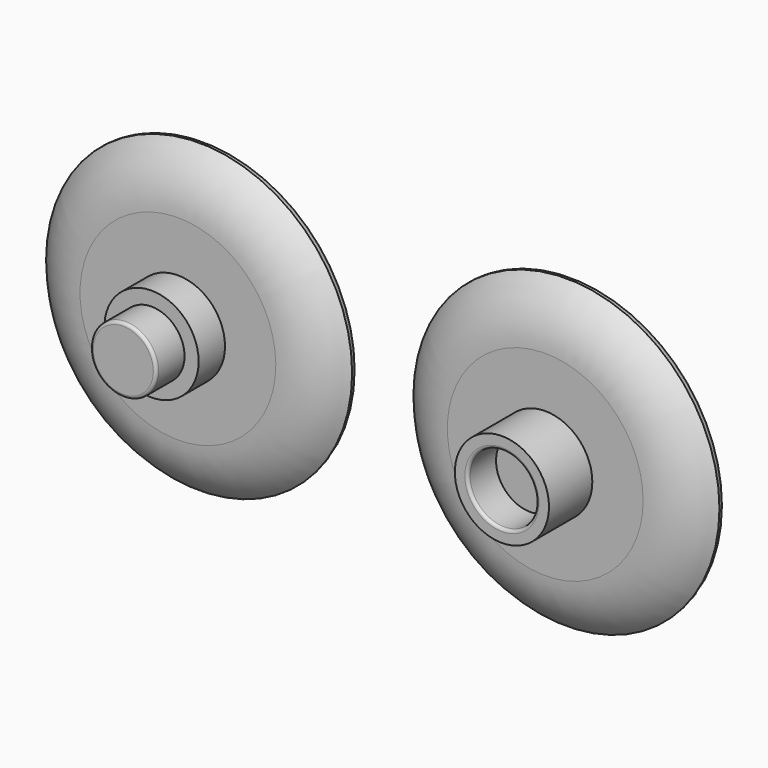
from build123d import *

# Parameters (mm, degrees)
F0_R      = 13
F1_DEPTH  = 3
F2_R      = 4
F3_DEPTH  = 2.8
F4_R      = 2.8
F5_DEPTH  = 3
F6_R      = 13
F7_DEPTH  = 3
F8_R      = 4
F9_DEPTH  = 4.6
F10_R     = 2.9
F11_DEPTH = 3
F12_R     = 0.75
F12_2_R   = 0.75
F13_R     = 0.25
F13_2_R   = 0.25


# Not quite as in the source:
# - a fillet or chamfer that OpenCascade refuses, or shapes differently, is made with other operations: its cross-section is extruded or revolved along the edge and cut away or added


with BuildPart() as f1:
    # F0 (on Front) → F1 (new body)
    with BuildSketch(Plane.XZ):
        Circle(F0_R)
    extrude(amount=F1_DEPTH)

    # F2 (on face) → F3 (join)
    with BuildSketch(Plane.XZ.offset(3)):
        Circle(F2_R)
    extrude(amount=F3_DEPTH)

    # F4 (on face) → F5 (join)
    with BuildSketch(Plane.XZ.offset(5.8)):
        Circle(F4_R)
    extrude(amount=F5_DEPTH)

    # F12
    f12_edges = [f1.edges().sort_by_distance(p)[0] for p in [
        (-13, 0, 0),
    ]]
    fillet(f12_edges, radius=F12_R)

    # F13
    f13_edges = [f1.edges().sort_by_distance(p)[0] for p in [
        (-2.8, -8.8, 0),
    ]]
    fillet(f13_edges, radius=F13_R)

    # F14: fillet of radius 6 on 1 edges, made by hand

    # F14_s1 → F14_t2 (revolve, cut)
    with BuildSketch(Plane.XY):
        with BuildLine():
            ThreePointArc((8.3162515012, -3), (10.9143277126, -2.4083269132), (13, -0.75))
            Line((13, -0.75), (13, -3))
            Line((13, -3), (8.3162515012, -3))
        make_face()
    revolve(axis=Axis((0, -3, 0), (0, -1, 0)), mode=Mode.SUBTRACT)


with BuildPart() as f7:
    # F6 (on Front) → F7 (new body)
    with BuildSketch(Plane.XZ):
        with Locations((31.2039515188, 0)):
            Circle(F6_R)
    extrude(amount=F7_DEPTH)

    # F8 (on face) → F9 (join)
    with BuildSketch(Plane.XZ.offset(3)):
        with Locations((31.2039515188, 0)):
            Circle(F8_R)
    extrude(amount=F9_DEPTH)

    # F10 (on face) → F11 (cut)
    with BuildSketch(Plane.XZ.offset(7.6)):
        with Locations((31.2039515188, 0)):
            Circle(F10_R)
    extrude(amount=-F11_DEPTH, mode=Mode.SUBTRACT)

    # F12#2
    f12_2_edges = [f7.edges().sort_by_distance(p)[0] for p in [
        (18.203952, 0, 0),
    ]]
    fillet(f12_2_edges, radius=F12_2_R)

    # F13#2
    f13_2_edges = [f7.edges().sort_by_distance(p)[0] for p in [
        (28.303952, -7.6, 0),
    ]]
    fillet(f13_2_edges, radius=F13_2_R)

    # F14#2: fillet of radius 6 on 1 edges, made by hand

    # F14_2_s1 → F14_2_t2 (revolve, cut)
    with BuildSketch(Plane.XY):
        with BuildLine():
            ThreePointArc((39.52020302, -3), (42.1182792313, -2.4083269132), (44.2039515188, -0.75))
            Line((44.2039515188, -0.75), (44.2039515188, -3))
            Line((44.2039515188, -3), (39.52020302, -3))
        make_face()
    revolve(axis=Axis((31.2039515188, -3, 0), (0, -1, 0)), mode=Mode.SUBTRACT)


solid = Compound([f1.part, f7.part])
